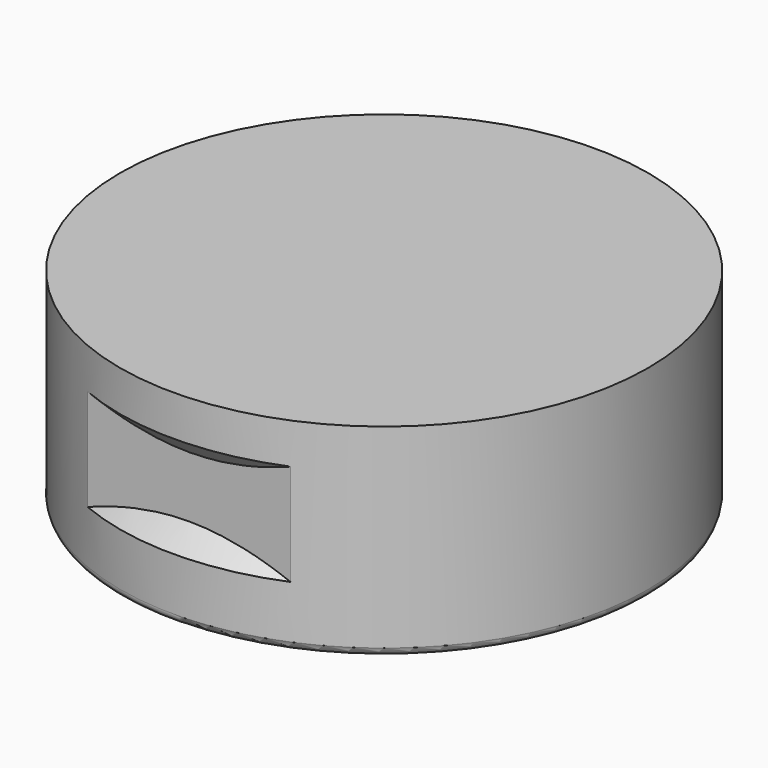
from build123d import *

# Parameters (mm, degrees)
F0_R     = 65
F1_DEPTH = 50
F2_R     = 2
F4_W     = 50
F4_H     = 15
F5_DEPTH = 25
F6_SIZE  = 4.99999


# Not quite as in the source:
# - a fillet or chamfer is up to 0.001 mm smaller than in the source, because OpenCascade refuses the exact size


with BuildPart() as f1:
    # F0 (on Top) → F1 (new body)
    with BuildSketch(Plane.XY):
        Circle(F0_R)
    extrude(amount=F1_DEPTH)

    # F2
    f2_edges = [f1.edges().sort_by_distance(p)[0] for p in [
        (-65, 0, 0),
    ]]
    fillet(f2_edges, radius=F2_R)

    # F4 (on offset) → F5 (cut)
    with BuildSketch(Plane.XZ.offset(60)):
        with Locations((0, 27.5)):
            Rectangle(F4_W, F4_H)
    extrude(amount=F5_DEPTH, mode=Mode.SUBTRACT)

    # F6 (size 5 in the source; OpenCascade refuses exactly that, so slightly less here)
    f6_edges = [f1.edges().sort_by_distance(p)[0] for p in [
        (0, -65, 20),
        (0, -65, 35),
    ]]
    chamfer(f6_edges, length=F6_SIZE)


solid = f1.part
